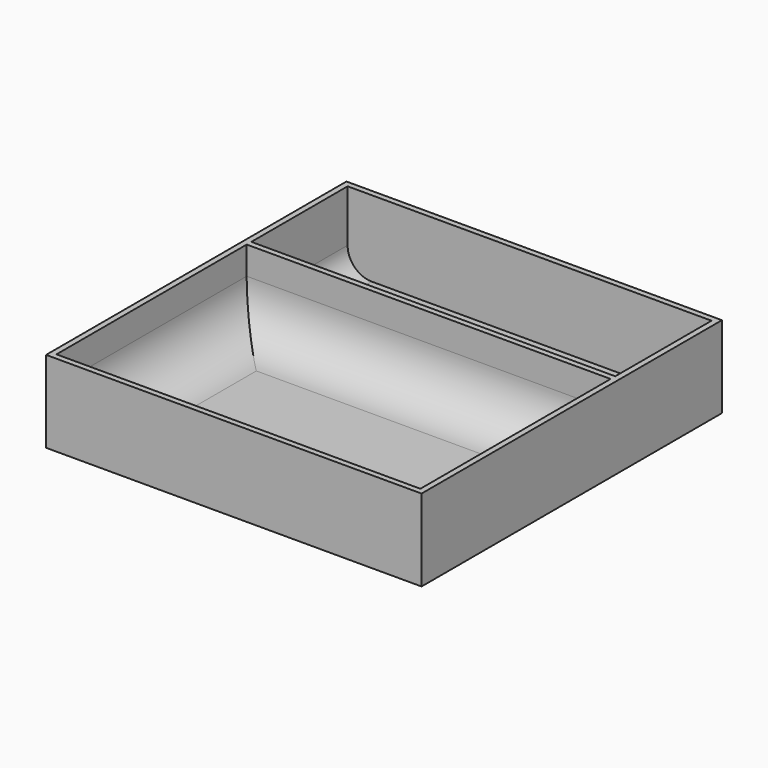
from build123d import *

# Parameters (mm, degrees)
F0_W     = 151.2
F0_H     = 50
F1_DEPTH = 2.4
F0_H_2   = 98.8
F0_W_2   = 156
F0_H_3   = 156
F0_H_4   = 2.4
F2_DEPTH = 34
F3_R     = 20
F4_R     = 10


with BuildPart() as f1:
    # F0 (on Top) → F1 (new body)
    with BuildSketch(Plane.XY):
        with Locations((0, 50.6)):
            Rectangle(F0_W, F0_H)
    extrude(amount=F1_DEPTH)



with BuildPart() as f1b:
    # F0 (on Top) → F1, piece 2 (new body)
    with BuildSketch(Plane.XY):
        with Locations((0, -26.2)):
            Rectangle(F0_W, F0_H_2)
    extrude(amount=F1_DEPTH)


with BuildPart() as f1_1:
    add(f1.part)

    add(f1b.part)  # F2 merges F1b
    # F0 (on Top) → F2 (join)
    with BuildSketch(Plane.XY):
        Rectangle(F0_W_2, F0_H_3)
        Polygon((-75.6, 25.6), (-75.6, 75.6), (75.6, 75.6), (75.6, 25.6), (75.6, 23.2), (75.6, -75.6), (-75.6, -75.6), (-75.6, 23.2), align=None, mode=Mode.SUBTRACT)
        with Locations((0, 24.4)):
            Rectangle(F0_W, F0_H_4)
    extrude(amount=F2_DEPTH)

    # F3
    f3_edges = [f1_1.edges().sort_by_distance(p)[0] for p in [
        (0, -75.6, 2.4),
        (75.6, -26.2, 2.4),
        (0, 23.2, 2.4),
        (-75.6, -26.2, 2.4),
    ]]
    fillet(f3_edges, radius=F3_R)

    # F4
    f4_edges = [f1_1.edges().sort_by_distance(p)[0] for p in [
        (75.6, 50.6, 2.4),
        (-75.6, 50.6, 2.4),
    ]]
    fillet(f4_edges, radius=F4_R)


solid = f1_1.part
